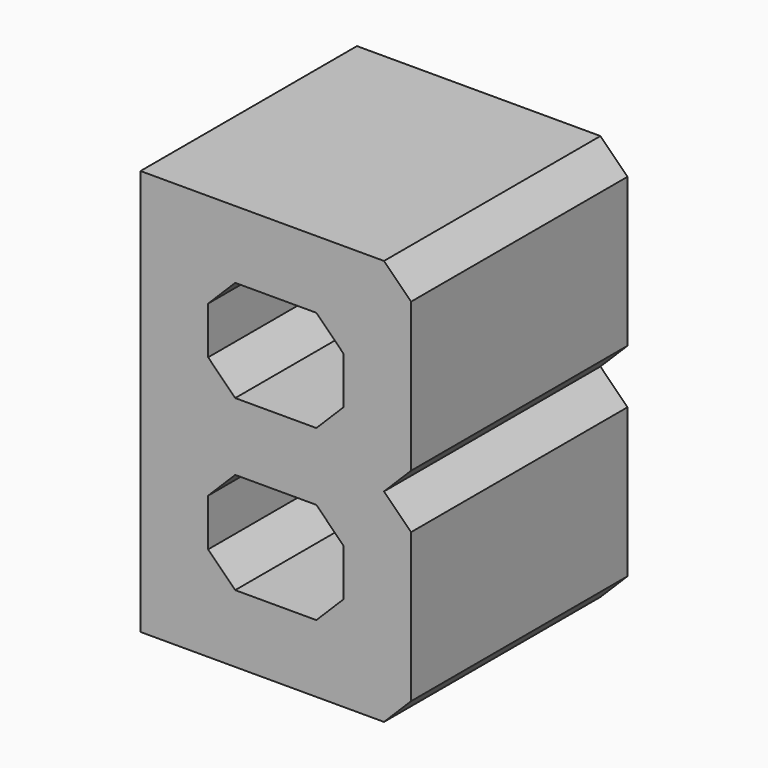
from build123d import *

# Parameters (mm, degrees)
F0_W     = 10
F0_H     = 7.5
F1_DEPTH = 20
F2_SIZE  = 2
F4_DEPTH = 25


# Not quite as in the source:
# - a feature names something its author has since deleted; it is built from what else it names


with BuildPart() as f1:
    # F0 (on Front) → F1 (new body)
    with BuildSketch(Plane.XZ):
        Polygon((20, 30), (0, 30), (0, 0), (20, 0), (20, 15), align=None)
        with Locations((10, 8.75)):
            Rectangle(F0_W, F0_H, mode=Mode.SUBTRACT)
        with Locations((10, 21.25)):
            Rectangle(F0_W, F0_H, mode=Mode.SUBTRACT)
    extrude(amount=F1_DEPTH)

    # F2
    f2_edges = [f1.edges().sort_by_distance(p)[0] for p in [
        (20, -10, 30),
        (5, -10, 17.5),
        (5, -10, 25),
        (5, -10, 12.5),
        (5, -10, 5),
        (15, -10, 25),
        (15, -10, 17.5),
        (15, -10, 12.5),
        (15, -10, 5),
        (20, -10, 0),
    ]]
    chamfer(f2_edges, length=F2_SIZE)

    # F3 (on face) → F4 (cut)
    with BuildSketch(Plane.XZ.offset(20)):
        Polygon((20, 13), (20, 15), (18, 15), align=None)
        Polygon((18, 15), (20, 15), (20, 17), align=None)
    extrude(amount=-F4_DEPTH, mode=Mode.SUBTRACT)


solid = f1.part
